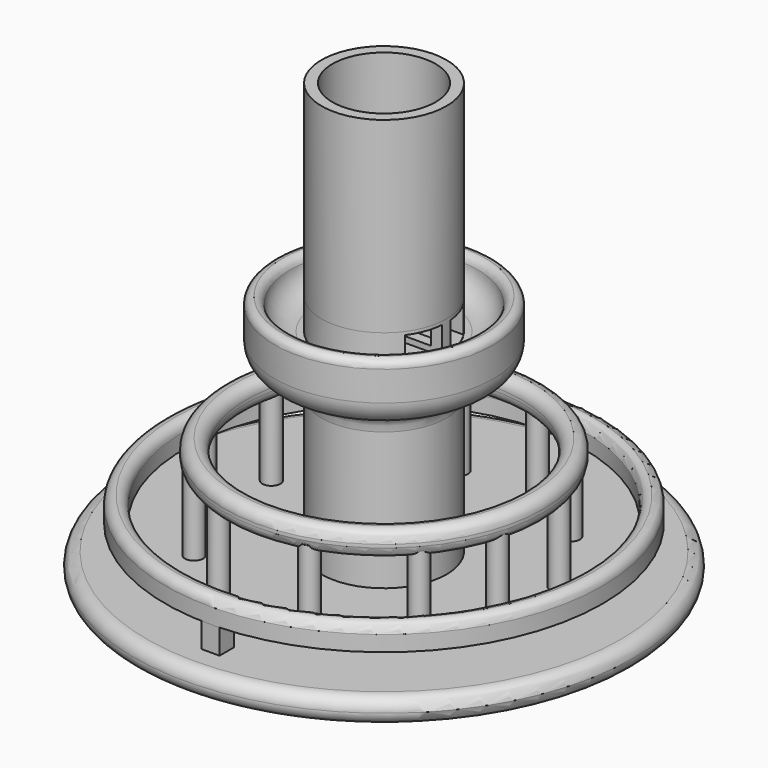
from build123d import *

# Parameters (mm, degrees)
F0_R      = 50.8
F1_DEPTH  = 5.08
F2_R      = 2.53999
F3_R      = 12.7
F4_DEPTH  = 88.9
F6_START  = 38.1
F5_R      = 22.225
F6_DEPTH  = 12.7
F7_R      = 5.08
F8_R      = 19.05
F8_R_2    = 12.7
F9_DEPTH  = 6.35
F10_R     = 5.08
F11_W     = 5.7031868491
F11_H     = 5.6271441281
F11_W_2   = 6.3115260564
F11_H_2   = 5.5511035025
F12_DEPTH = 12.7
F13_W     = 6.40402094
F13_H     = 5.6271441281
F13_W_2   = 5.8219179045
F13_H_2   = 5.6150481105
F14_DEPTH = 12.7
F15_R     = 10.4977096987
F16_DEPTH = 43.18
F17_R     = 1.574799746
F19_START = 20.32
F18_R     = 32.385
F18_R_2   = 27.94
F19_DEPTH = 5.08
F20_R     = 2.22249
F21_R     = 1.8418202524
F22_DEPTH = 21.59
F24_START = 10.16
F23_R     = 44.45
F23_R_2   = 40.64
F24_DEPTH = 5.08
F25_R     = 1.90499
F26_R     = 5.08
F28_START = 5.08
F27_W     = 3.6266420502
F27_H     = 3.635276109
F28_DEPTH = 5.08


# Not quite as in the source:
# - a fillet or chamfer is up to 0.001 mm smaller than in the source, because OpenCascade refuses the exact size


with BuildPart() as f1:
    # F0 (on Top) → F1 (new body)
    with BuildSketch(Plane.XY):
        Circle(F0_R)
    extrude(amount=F1_DEPTH)

    # F2 (radius 2.54 in the source; OpenCascade refuses exactly that, so slightly less here)
    f2_edges = [f1.edges().sort_by_distance(p)[0] for p in [
        (50.8, 0, 2.54),
        (-50.8, 0, 0),
        (-50.8, 0, 5.08),
    ]]
    fillet(f2_edges, radius=F2_R)

    # F3 (on Top) → F4 (join)
    with BuildSketch(Plane.XY):
        Circle(F3_R)
    extrude(amount=F4_DEPTH)

    # F5 (on Top) → F6 (join)
    with BuildSketch(Plane.XY.offset(F6_START)):
        Circle(F5_R)
    extrude(amount=F6_DEPTH)

    # F7
    f7_edges = [f1.edges().sort_by_distance(p)[0] for p in [
        (-22.225, 0, 38.1),
    ]]
    fillet(f7_edges, radius=F7_R)

    # F8 (on face) → F9 (cut)
    with BuildSketch(Plane.XY.offset(50.8)):
        Circle(F8_R)
        Circle(F8_R_2, mode=Mode.SUBTRACT)
    extrude(amount=-F9_DEPTH, mode=Mode.SUBTRACT)

    # F10
    f10_edges = [f1.edges().sort_by_distance(p)[0] for p in [
        (-19.05, 0, 44.45),
    ]]
    fillet(f10_edges, radius=F10_R)

    # F11 (on Right) → F12 (cut)
    with BuildSketch(Plane.YZ):
        with Locations((-5.325405742, 47.4032554775)):
            Rectangle(F11_W, F11_H)
        with Locations((5.2445002366, 47.4412757903)):
            Rectangle(F11_W_2, F11_H_2)
    extrude(amount=-F12_DEPTH, mode=Mode.SUBTRACT)

    # F13 (on Right) → F14 (cut)
    with BuildSketch(Plane.YZ):
        with Locations((-4.3034976698, 47.3379362375)):
            Rectangle(F13_W, F13_H)
        with Locations((3.9530118229, 47.3439842463)):
            Rectangle(F13_W_2, F13_H_2)
    extrude(amount=F14_DEPTH, mode=Mode.SUBTRACT)

    # F15 (on face) → F16 (cut)
    with BuildSketch(Plane.XY.offset(88.9)):
        Circle(F15_R)
    extrude(amount=-F16_DEPTH, mode=Mode.SUBTRACT)

    # F17
    f17_edges = [f1.edges().sort_by_distance(p)[0] for p in [
        (-19.05, 0, 50.8),
        (-22.225, 0, 50.8),
    ]]
    fillet(f17_edges, radius=F17_R)

    # F26
    f26_edges = [f1.edges().sort_by_distance(p)[0] for p in [
        (-12.7, 0, 38.1),
    ]]
    fillet(f26_edges, radius=F26_R)


with BuildPart() as f19:
    # F18 (on Top) → F19 (new body)
    with BuildSketch(Plane.XY.offset(F19_START)):
        Circle(F18_R)
        Circle(F18_R_2, mode=Mode.SUBTRACT)
    extrude(amount=F19_DEPTH)

    # F20 (radius 2.2225 in the source; OpenCascade refuses exactly that, so slightly less here)
    f20_edges = [f19.edges().sort_by_distance(p)[0] for p in [
        (-27.94, 0, 25.4),
        (-32.385, 0, 25.4),
        (-27.94, 0, 20.32),
        (-32.385, 0, 20.32),
    ]]
    fillet(f20_edges, radius=F20_R)


with BuildPart() as f22:
    # F21 (on Top) → F22 (new body)
    with BuildSketch(Plane.XY):
        with Locations((-11.4090433344, -27.8096720576)):
            Circle(F21_R)
    extrude(amount=F22_DEPTH)


with BuildPart() as f22b:
    # F21 (on Top) → F22, piece 2 (new body)
    with BuildSketch(Plane.XY):
        with Locations((8.1535298377, -29.0949922055)):
            Circle(F21_R)
    extrude(amount=F22_DEPTH)


with BuildPart() as f22c:
    # F21 (on Top) → F22, piece 3 (new body)
    with BuildSketch(Plane.XY):
        with Locations((22.8778347373, -19.703803584)):
            Circle(F21_R)
    extrude(amount=F22_DEPTH)


with BuildPart() as f22d:
    # F21 (on Top) → F22, piece 4 (new body)
    with BuildSketch(Plane.XY):
        with Locations((-22.6929332038, -19.9089368758)):
            Circle(F21_R)
    extrude(amount=F22_DEPTH)


with BuildPart() as f22e:
    # F21 (on Top) → F22, piece 5 (new body)
    with BuildSketch(Plane.XY):
        with Locations((29.2916446924, -7.8023611568)):
            Circle(F21_R)
    extrude(amount=F22_DEPTH)


with BuildPart() as f22f:
    # F21 (on Top) → F22, piece 6 (new body)
    with BuildSketch(Plane.XY):
        with Locations((29.2916446924, 7.8731411513)):
            Circle(F21_R)
    extrude(amount=F22_DEPTH)


with BuildPart() as f22g:
    # F21 (on Top) → F22, piece 7 (new body)
    with BuildSketch(Plane.XY):
        with Locations((19.9004560709, 22.5974460508)):
            Circle(F21_R)
    extrude(amount=F22_DEPTH)


with BuildPart() as f22h:
    # F21 (on Top) → F22, piece 8 (new body)
    with BuildSketch(Plane.XY):
        with Locations((7.9990136437, 29.011256006)):
            Circle(F21_R)
    extrude(amount=F22_DEPTH)


with BuildPart() as f22i:
    # F21 (on Top) → F22, piece 9 (new body)
    with BuildSketch(Plane.XY):
        with Locations((-8.0465003848, 29.1461069137)):
            Circle(F21_R)
    extrude(amount=F22_DEPTH)


with BuildPart() as f22j:
    # F21 (on Top) → F22, piece 10 (new body)
    with BuildSketch(Plane.XY):
        with Locations((-22.7708052844, 19.7549182922)):
            Circle(F21_R)
    extrude(amount=F22_DEPTH)


with BuildPart() as f22k:
    # F21 (on Top) → F22, piece 11 (new body)
    with BuildSketch(Plane.XY):
        with Locations((-29.1846152395, 7.853475865)):
            Circle(F21_R)
    extrude(amount=F22_DEPTH)


with BuildPart() as f22l:
    # F21 (on Top) → F22, piece 12 (new body)
    with BuildSketch(Plane.XY):
        with Locations((-28.4910995079, -9.9379075691)):
            Circle(F21_R)
    extrude(amount=F22_DEPTH)


with BuildPart() as f24:
    # F23 (on Top) → F24 (new body)
    with BuildSketch(Plane.XY.offset(F24_START)):
        Circle(F23_R)
        Circle(F23_R_2, mode=Mode.SUBTRACT)
    extrude(amount=F24_DEPTH)

    # F25 (radius 1.905 in the source; OpenCascade refuses exactly that, so slightly less here)
    f25_edges = [f24.edges().sort_by_distance(p)[0] for p in [
        (-40.64, 0, 15.24),
        (-44.45, 0, 15.24),
    ]]
    fillet(f25_edges, radius=F25_R)


with BuildPart() as f28:
    # F27 (on Top) → F28 (new body)
    with BuildSketch(Plane.XY.offset(F28_START)):
        with Locations((0.2091563074, -42.5092149526)):
            Rectangle(F27_W, F27_H)
    extrude(amount=F28_DEPTH)


solid = Compound([f1.part, f19.part, f22.part, f22b.part, f22c.part, f22d.part, f22e.part, f22f.part, f22g.part, f22h.part, f22i.part, f22j.part, f22k.part, f22l.part, f24.part, f28.part])
